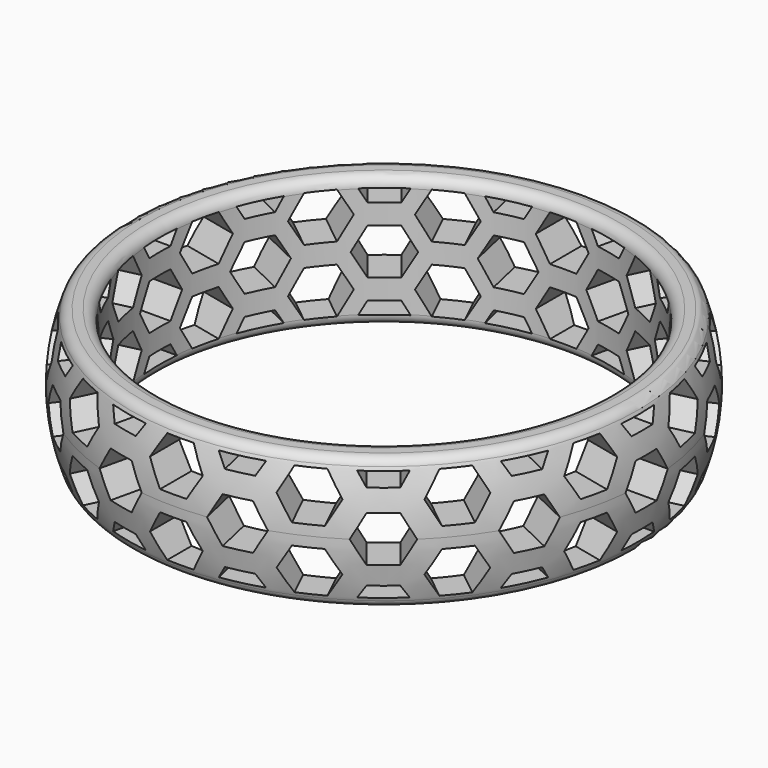
from build123d import *

# Parameters (mm, degrees)
F0_R      = 127
F1_DEPTH  = 63.5
F2_R      = 107.95
F3_DEPTH  = 254
F6_DEPTH  = 127.001
F7_COUNT  = 14
F13_DEPTH = 190.5
F14_COUNT = 14


# Not quite as in the source:
# - a fillet or chamfer that OpenCascade refuses, or shapes differently, is made with other operations: its cross-section is extruded or revolved along the edge and cut away or added


with BuildPart() as f1:
    # F0 (on Top) → F1 (new body)
    with BuildSketch(Plane.XY):
        Circle(F0_R)
    extrude(amount=F1_DEPTH)

    # F2 (on face) → F3 (cut)
    with BuildSketch(Plane.XY.offset(63.5)):
        Circle(F2_R)
    extrude(amount=-F3_DEPTH, mode=Mode.SUBTRACT)

    # F5 (on Front) → F6 (cut, through all)
    with BuildSketch(Plane.XZ):
        Polygon((6.35, 36.6264773719), (12.7, 47.625), (6.35, 58.6235226281), (-6.35, 58.6235226281), (-12.7, 47.625), (-6.35, 36.6264773719), align=None)
        Polygon((-12.7, 15.875), (-6.35, 4.8764773719), (6.35, 4.8764773719), (12.7, 15.875), (6.35, 26.8735226281), (-6.35, 26.8735226281), align=None)
    f6 = extrude(amount=F6_DEPTH, mode=Mode.SUBTRACT)

    # F7: F6 ×14 about axis
    f7_axis = Axis((0, 0, 31.75), (0, 0, 1))
    for i in range(1, F7_COUNT):
        add(f6.rotate(f7_axis, i * 360 / F7_COUNT), mode=Mode.SUBTRACT)

    # F11 (on line) → F13 (cut, symmetric)
    with BuildSketch(Plane(origin=(108.174677984, 52.0941793148, 0), x_dir=(0.4338837391, -0.9009688679, 0), z_dir=(-0.9009688679, -0.4338837391, 0))):
        Polygon((-6.35, 42.7485226281), (-12.7, 31.75), (-6.35, 20.7514773719), (6.35, 20.7514773719), (12.7, 31.75), (6.35, 42.7485226281), align=None)
        Polygon((-9.8845644766, 58.6235226281), (-6.35, 52.5014773719), (6.35, 52.5014773719), (9.8845644766, 58.6235226281), align=None)
        Polygon((9.8845644766, 4.8764773719), (6.35, 10.9985226281), (-6.35, 10.9985226281), (-9.8845644766, 4.8764773719), align=None)
    f13 = extrude(amount=F13_DEPTH, both=True, mode=Mode.SUBTRACT)

    # F14: F13 ×14 about axis
    f14_axis = Axis((0, 0, 46.8367896974), (0, 0, 1))
    for i in range(1, F14_COUNT):
        add(f13.rotate(f14_axis, i * 360 / F14_COUNT), mode=Mode.SUBTRACT)

    # F15 (on Right) → F16 (revolve, cut)
    with BuildSketch(Plane.YZ):
        with BuildLine():
            Line((120.65, 0), (127, 0))
            Line((127, 0), (127, 31.7500008503))
            ThreePointArc((127, 31.7500008503), (125.3969348617, 15.5606134612), (120.65, 0))
        make_face()
        with BuildLine():
            ThreePointArc((120.65, 63.5), (125.3969346949, 47.9393873725), (127, 31.7500008503))
            Line((127, 31.7500008503), (127, 63.5))
            Line((127, 63.5), (120.65, 63.5))
        make_face()
    revolve(axis=Axis((0, 0, 31.75), (0, 0, 1)), mode=Mode.SUBTRACT)

    # F17: fillet of radius 5.08 on 4 edges, made by hand

    # F17_s1 → F17_t2 (revolve, cut)
    with BuildSketch(Plane.XZ):
        with BuildLine():
            ThreePointArc((113.03, 63.5), (109.4378975516, 62.0121024484), (107.95, 58.42))
            Line((107.95, 58.42), (107.95, 63.5))
            Line((107.95, 63.5), (113.03, 63.5))
        make_face()
    revolve(axis=Axis((0, 0, 63.5), (0, 0, 1)), mode=Mode.SUBTRACT)

    # F17_s3 → F17_t4 (revolve, cut)
    with BuildSketch(Plane.XZ):
        with BuildLine():
            ThreePointArc((113.03, 0), (109.4378975516, 1.4878975516), (107.95, 5.08))
            Line((107.95, 5.08), (107.95, 0))
            Line((107.95, 0), (113.03, 0))
        make_face()
    revolve(axis=Axis((0, 0, 0), (0, 0, 1)), mode=Mode.SUBTRACT)

    # F17_s5 → F17_t6 (revolve, cut)
    with BuildSketch(Plane.YZ):
        with BuildLine():
            ThreePointArc((121.9540084442, 60.168852459), (120.0933305398, 62.5847671299), (117.1845310014, 63.5))
            Line((117.1845310014, 63.5), (120.65, 63.5))
            ThreePointArc((120.65, 63.5), (121.320050663, 61.8414906753), (121.9540084442, 60.168852459))
        make_face()
    revolve(axis=Axis((0, 0, 63.5), (0, 0, 1)), mode=Mode.SUBTRACT)

    # F17_s7 → F17_t8 (revolve, cut)
    with BuildSketch(Plane.YZ):
        with BuildLine():
            ThreePointArc((121.9540084442, 3.331147541), (120.0933305398, 0.9152328701), (117.1845310014, 0))
            Line((117.1845310014, 0), (120.65, 0))
            ThreePointArc((120.65, 0), (121.320050663, 1.6585093247), (121.9540084442, 3.331147541))
        make_face()
    revolve(axis=Axis((0, 0, 0), (0, 0, 1)), mode=Mode.SUBTRACT)


solid = f1.part
